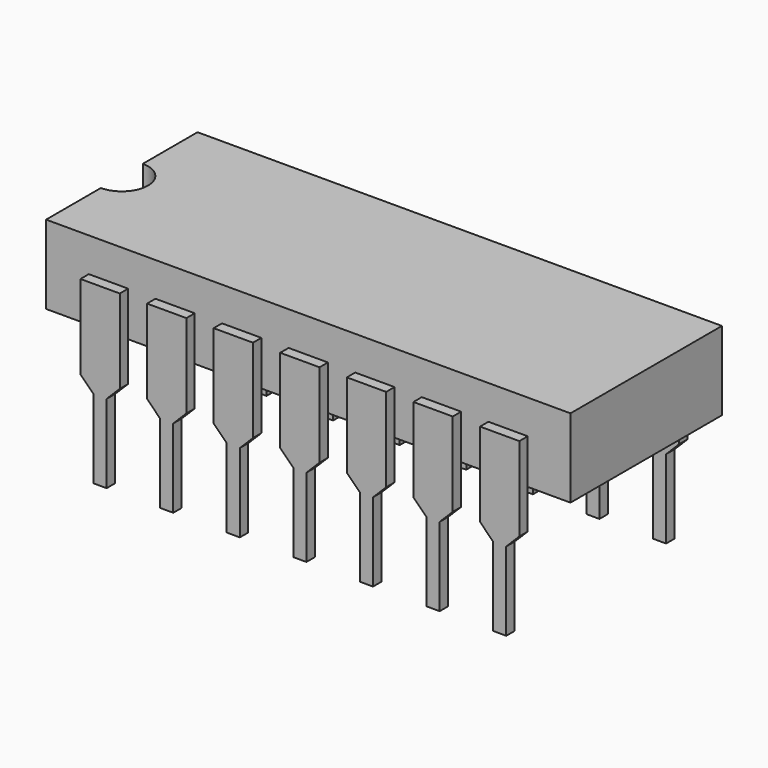
from build123d import *

# Parameters (mm, degrees)
F1_START = 2
F1_DEPTH = 3
F3_DEPTH = 0.4


# Not quite as in the source:
# - a pattern or mirror of a feature is missing from the dataset's text; its kind, count and spacing are read off the source's solid


with BuildPart() as f1:
    # F0 (on Top) → F1 (new body)
    with BuildSketch(Plane.XY.offset(F1_START)):
        with BuildLine():
            Line((10, 3.61), (-10, 3.61))
            Line((-10, 3.61), (-10, 1))
            ThreePointArc((-10, 1), (-9, 0), (-10, -1))
            Line((-10, -1), (-10, -3.61))
            Line((-10, -3.61), (10, -3.61))
            Line((10, -3.61), (10, 3.61))
        make_face()
    extrude(amount=F1_DEPTH)

    # F2 (on face) → F3 (join)
    with BuildSketch(Plane.XZ.offset(3.61)):
        Polygon((-6.87, 3.7), (-8.37, 3.7), (-8.37, 0.5), (-7.87, 0), (-7.87, -3), (-7.37, -3), (-7.37, 0), (-6.87, 0.5), align=None)
        Polygon((-5.83, 0.5), (-5.33, 0), (-5.33, -3), (-4.83, -3), (-4.83, 0), (-4.33, 0.5), (-4.33, 3.7), (-5.83, 3.7), align=None)
        Polygon((-3.29, 0.5), (-2.79, 0), (-2.79, -3), (-2.29, -3), (-2.29, 0), (-1.79, 0.5), (-1.79, 3.7), (-3.29, 3.7), align=None)
        Polygon((-0.75, 0.5), (-0.25, 0), (-0.25, -3), (0.25, -3), (0.25, 0), (0.75, 0.5), (0.75, 3.7), (-0.75, 3.7), align=None)
        Polygon((1.79, 0.5), (2.29, 0), (2.29, -3), (2.79, -3), (2.79, 0), (3.29, 0.5), (3.29, 3.7), (1.79, 3.7), align=None)
        Polygon((4.33, 0.5), (4.83, 0), (4.83, -3), (5.33, -3), (5.33, 0), (5.83, 0.5), (5.83, 3.7), (4.33, 3.7), align=None)
        Polygon((6.87, 0.5), (7.37, 0), (7.37, -3), (7.87, -3), (7.87, 0), (8.37, 0.5), (8.37, 3.7), (6.87, 3.7), align=None)
    f3 = extrude(amount=F3_DEPTH)

    # F3_copies: F3 across plane
    add(f3.mirror(Plane.ZX))


solid = f1.part
